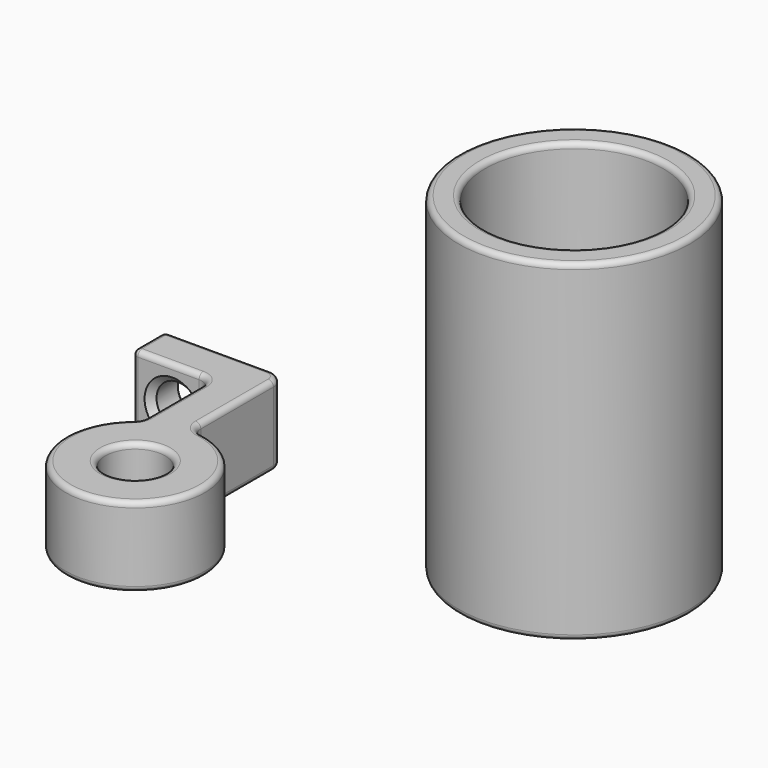
from build123d import *

# Parameters (mm, degrees)
F0_R     = 2.25
F1_DEPTH = 6
F2_R     = 1.6
F3_DEPTH = 3.001
F4_SIZE  = 0.5
F5_R     = 1
F6_R     = 0.4
F0_R_2   = 8.7
F0_R_3   = 6.7
F7_DEPTH = 25
F8_DEPTH = 2
F9_R     = 0.4


# Not quite as in the source:
# - a feature names something its author has since deleted; it is built from what else it names


with BuildPart() as f1:
    # F0 (on Top) → F1 (new body)
    with BuildSketch(Plane.XY):
        with BuildLine():
            Line((9, 0), (0, 0))
            Line((0, 0), (0, -3))
            Line((0, -3), (6, -3))
            Line((6, -3), (6, -9.6915780151))
            ThreePointArc((6, -9.6915780151), (10.5721457597, -19.0090775309), (9, -8.75))
            Line((9, -8.75), (9, 0))
        make_face()
        with Locations((9, -14)):
            Circle(F0_R, mode=Mode.SUBTRACT)
    extrude(amount=F1_DEPTH)

    # F2 (on face) → F3 (cut, through all)
    with BuildSketch(Plane.XZ.offset(3)):
        with Locations((3, 3)):
            Circle(F2_R)
    extrude(amount=-F3_DEPTH, mode=Mode.SUBTRACT)

    # F4
    f4_edges = [f1.edges().sort_by_distance(p)[0] for p in [
        (1.4, -3, 3),
        (1.4, 0, 3),
    ]]
    chamfer(f4_edges, length=F4_SIZE)

    # F5
    f5_edges = [f1.edges().sort_by_distance(p)[0] for p in [
        (6, -3, 3),
        (9, 0, 3),
        (9, -8.75, 3),
        (6, -9.691578, 3),
    ]]
    fillet(f5_edges, radius=F5_R)

    # F6
    f6_edges = [f1.edges().sort_by_distance(p)[0] for p in [
        (9, -4.415259, 6),
        (9.238423, -8.478593, 6),
        (8.707107, -0.292893, 6),
        (10.384667, -19.064109, 6),
        (4, 0, 6),
        (5.905539, -9.621921, 6),
        (0, -1.5, 6),
        (6, -6.598828, 6),
        (2.5, -3, 6),
        (5.707107, -3.292893, 6),
        (6.75, -14, 6),
        (9, -4.415259, 0),
        (9.238423, -8.478593, 0),
        (8.707107, -0.292893, 0),
        (10.384667, -19.064109, 0),
        (4, 0, 0),
        (5.905539, -9.621921, 0),
        (0, -1.5, 0),
        (6, -6.598828, 0),
        (2.5, -3, 0),
        (5.707107, -3.292893, 0),
        (6.75, -14, 0),
        (0, 0, 3),
        (0, -3, 3),
    ]]
    fillet(f6_edges, radius=F6_R)


with BuildPart() as f7:
    # F0 (on Top) → F7 (new body)
    with BuildSketch(Plane.XY):
        with Locations((30.8381635696, 0)):
            Circle(F0_R_2)
        with Locations((30.8381635696, 0)):
            Circle(F0_R_3, mode=Mode.SUBTRACT)
    extrude(amount=F7_DEPTH)

    # F0 (on Top) → F8 (join)
    with BuildSketch(Plane.XY):
        with Locations((30.8381635696, 0)):
            Circle(F0_R_3)
        with Locations((30.8381635696, 0)):
            Circle(F0_R, mode=Mode.SUBTRACT)
    extrude(amount=F8_DEPTH)

    # F9
    f9_edges = [f7.edges().sort_by_distance(p)[0] for p in [
        (22.138164, 0, 0),
        (28.588164, 0, 0),
        (24.138164, 0, 2),
        (28.588164, 0, 2),
        (22.138164, 0, 25),
        (24.138164, 0, 25),
    ]]
    fillet(f9_edges, radius=F9_R)


solid = Compound([f1.part, f7.part])
